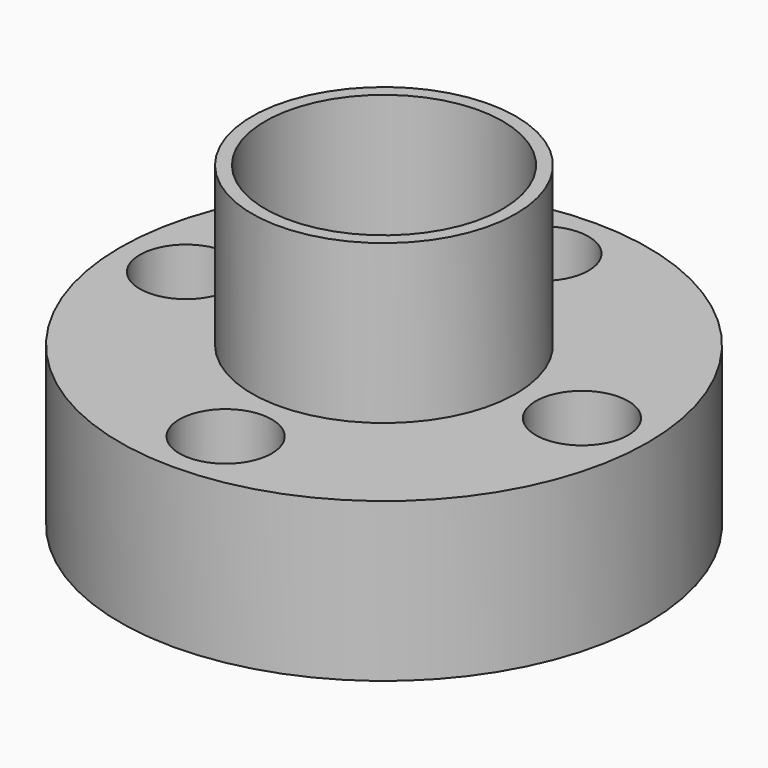
from build123d import *

# Parameters (mm, degrees)
F1_R     = 10
F2_DEPTH = 6
F0_R     = 5
F0_R_2   = 4.5
F0_R_3   = 1.75
F3_DEPTH = 6
F4_DEPTH = 6
F7_DEPTH = 12


# Not quite as in the source:
# - the program builds the solid bodies; features that only make, move or delete a surface that nothing else refers to are left out


with BuildPart() as f2:
    # F1 (on Top) → F2 (new body)
    with BuildSketch(Plane.XY):
        Circle(F1_R)
    extrude(amount=F2_DEPTH)

    # F0 (on Top) → F3 (cut, symmetric)
    with BuildSketch(Plane.XY):
        Circle(F0_R)
        Circle(F0_R_2, mode=Mode.SUBTRACT)
        with Locations((0, 7.5)):
            Circle(F0_R_3)
        with Locations((-7.5, 0)):
            Circle(F0_R_3)
        with Locations((0, -7.5)):
            Circle(F0_R_3)
        with Locations((7.5, 0)):
            Circle(F0_R_3)
    extrude(amount=F3_DEPTH, both=True, mode=Mode.SUBTRACT)

    # F4 (cut): a face of the model
    f4_faces = [f2.faces().sort_by_distance(p)[0] for p in [
        (0, 0, 6),
    ]]
    extrude(f4_faces, amount=-F4_DEPTH, mode=Mode.SUBTRACT)

    # F0 (on Top) → F7 (join)
    with BuildSketch(Plane.XY):
        Circle(F0_R)
        Circle(F0_R_2, mode=Mode.SUBTRACT)
    extrude(amount=F7_DEPTH)


solid = f2.part
